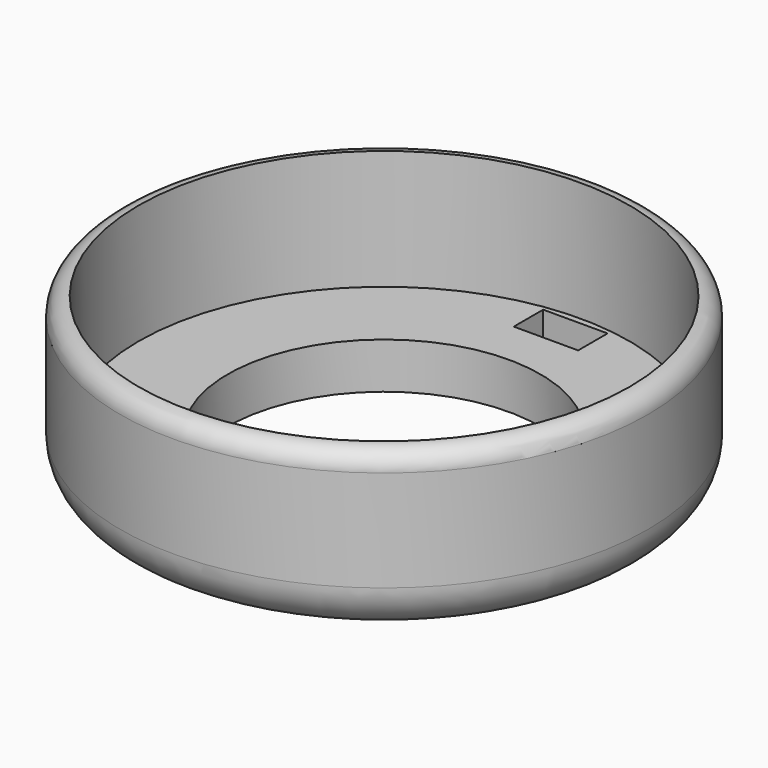
from build123d import *

# Parameters (mm, degrees)
F0_R     = 28.7
F0_R_2   = 26.7
F1_DEPTH = 18
F2_R     = 26.7
F3_DEPTH = 13
F4_R     = 17
F4_W     = 7
F4_H     = 4
F5_DEPTH = 5.001
F7_R     = 1.99999
F8_R     = 8.5
F8_R_2   = 6.5
F9_DEPTH = 2


# Not quite as in the source:
# - a fillet or chamfer that OpenCascade refuses, or shapes differently, is made with other operations: its cross-section is extruded or revolved along the edge and cut away or added
# - a fillet or chamfer is up to 0.001 mm smaller than in the source, because OpenCascade refuses the exact size


with BuildPart() as f1:
    # F0 (on Top) → F1 (new body)
    with BuildSketch(Plane.XY):
        Circle(F0_R)
        Circle(F0_R_2, mode=Mode.SUBTRACT)
        Circle(F0_R_2)
    extrude(amount=F1_DEPTH)

    # F2 (on face) → F3 (cut)
    with BuildSketch(Plane.XY.offset(18)):
        Circle(F2_R)
    extrude(amount=-F3_DEPTH, mode=Mode.SUBTRACT)

    # F4 (on face) → F5 (cut, through all)
    with BuildSketch(Plane.XY.offset(5)):
        Circle(F4_R)
        with Locations((0, 24)):
            Rectangle(F4_W, F4_H)
        Polygon((-20.8025588833, -7.9689110868), (-24.2666604984, -9.9689110868), (-20.7666604984, -16.0310889132), (-17.3025588833, -14.0310889132), align=None)
        Polygon((17.3025588833, -14.0310889132), (20.7666604984, -16.0310889132), (24.2666604984, -9.9689110868), (20.8025588833, -7.9689110868), align=None)
    extrude(amount=-F5_DEPTH, mode=Mode.SUBTRACT)

    # F6: fillet of radius 5 on 1 edges, made by hand

    # F6_s1 → F6_t2 (revolve, cut)
    with BuildSketch(Plane.XZ):
        with BuildLine():
            ThreePointArc((28.7, 5), (27.2355339059, 1.4644660941), (23.7, 0))
            Line((23.7, 0), (28.7, 0))
            Line((28.7, 0), (28.7, 5))
        make_face()
    revolve(axis=Axis((0, 0, 0), (0, 0, 1)), mode=Mode.SUBTRACT)

    # F7 (radius 2 in the source; OpenCascade refuses exactly that, so slightly less here)
    f7_edges = [f1.edges().sort_by_distance(p)[0] for p in [
        (-28.7, 0, 18),
    ]]
    fillet(f7_edges, radius=F7_R)

    # F8 (on Top) → F9 (join)
    with BuildSketch(Plane.XY):
        with Locations((0, 26)):
            Circle(F8_R)
        with Locations((0, 26)):
            Circle(F8_R_2, mode=Mode.SUBTRACT)
    extrude(amount=F9_DEPTH)


solid = f1.part
